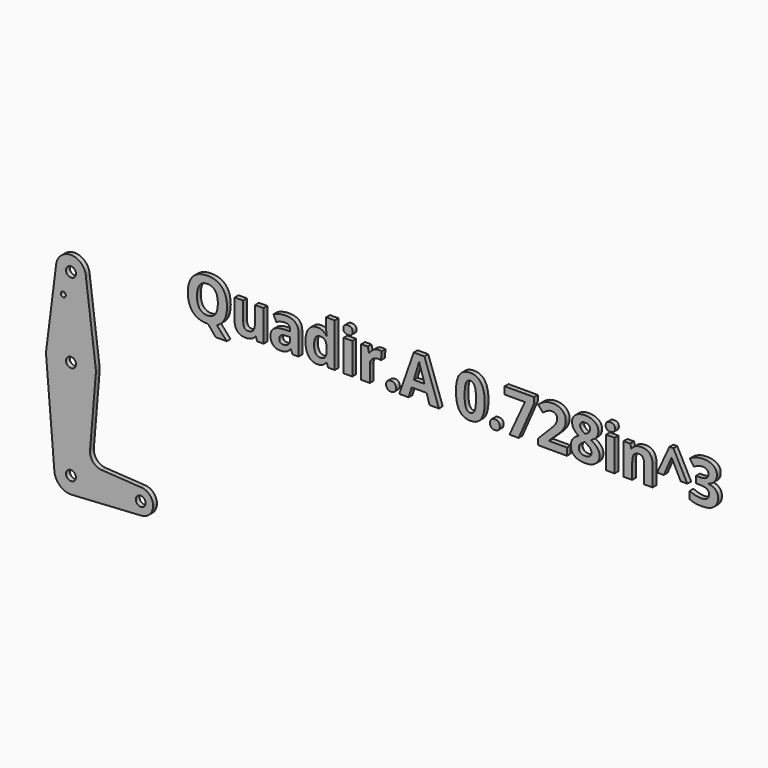
from build123d import *

# Parameters (mm, degrees)
F0_R         = 3.175
F0_R_2       = 1.5875
F0_R_3       = 3.1332260433
F0_R_4       = 3.1320796643
F0_TEXT_SIZE = 36.6663353311
F1_DEPTH     = 3.048


# Not quite as in the source:
# - Text() gives the source's letters only with a copy of the font that has no kerning and outlines rounded to 1/6400 em; it was checked with that copy


with BuildPart() as f1:
    # F0 (on Front) → F1 (new body)
    with BuildSketch(Plane.XZ):
        with BuildLine():
            ThreePointArc((-39.3125587135, 78.4643656567), (-30.4570816653, 67.7700037653), (-20.3369320583, 77.2763922459))
            ThreePointArc((-20.3369320583, 77.2763922459), (-20.3403427357, 77.5312682375), (-20.3505723252, 77.7859616989))
            ThreePointArc((-20.3505723252, 77.7859616989), (-29.521373533, 86.7953021042), (-39.3125587135, 78.4643656567))
        make_face()
        with Locations((-29.8619320583, 77.2763922459)):
            Circle(F0_R, mode=Mode.SUBTRACT)
        with BuildLine():
            ThreePointArc((-20.3505723252, 77.7859616989), (-20.3403427357, 77.5312682375), (-20.3369320583, 77.2763922459))
            ThreePointArc((-20.3369320583, 77.2763922459), (-30.4570816653, 67.7700037653), (-39.3125587135, 78.4643656567))
            Line((-39.3125587135, 78.4643656567), (-45.5153906923, 29.1192804))
            ThreePointArc((-45.5153906923, 29.1192804), (-29.5330383504, 42.3479849174), (-14.1124253975, 28.468543079))
            Line((-14.1124253975, 28.468543079), (-20.3505723252, 77.7859616989))
        make_face()
        with Locations((-34.7417071462, 63.0015922459)):
            Circle(F0_R_2, mode=Mode.SUBTRACT)
        with BuildLine():
            Line((-14.1124253975, 24.4842414128), (-14.1124253975, 28.468543079))
            ThreePointArc((-14.1124253975, 28.468543079), (-29.5330383504, 42.3479849174), (-45.5153906923, 29.1192804))
            Line((-45.5153906923, 29.1192804), (-45.6824995011, 27.7898878824))
            ThreePointArc((-45.6824995011, 27.7898878824), (-45.7369320583, 26.4763922459), (-45.6824995011, 25.1628966095))
            ThreePointArc((-45.6824995011, 25.1628966095), (-30.2031147479, 10.6050589884), (-14.1124253975, 24.4842414128))
        make_face()
        with Locations((-29.8619320583, 26.4763922459)):
            Circle(F0_R, mode=Mode.SUBTRACT)
        with BuildLine():
            ThreePointArc((-13.9869320583, 26.4763922459), (-14.0183364557, 27.4744420342), (-14.1124253975, 28.468543079))
            Line((-14.1124253975, 28.468543079), (-14.1124253975, 24.4842414128))
            ThreePointArc((-14.1124253975, 24.4842414128), (-14.0183364557, 25.4783424576), (-13.9869320583, 26.4763922459))
        make_face()
        with BuildLine():
            Line((-45.6824995011, 27.7898878824), (-45.5153906923, 29.1192804))
            ThreePointArc((-45.5153906923, 29.1192804), (-45.6129764836, 28.4563479305), (-45.6824995011, 27.7898878824))
        make_face()
        with BuildLine():
            Line((-17.6998397607, -18.9681708504), (-14.1124253975, 24.4842414128))
            ThreePointArc((-14.1124253975, 24.4842414128), (-30.2031147479, 10.6050589884), (-45.6824995011, 25.1628966095))
            Line((-45.6824995011, 25.1628966095), (-40.53226543, -36.8697612897))
            ThreePointArc((-40.53226543, -36.8697612897), (-29.7850068275, -26.3524426112), (-19.1904896536, -37.0236077541))
            ThreePointArc((-19.1904896536, -37.0236077541), (-21.9201856875, -44.1516051993), (-28.7127914479, -47.6329978805))
            Line((-28.7127914479, -47.6329978805), (15.0742024143, -44.946207045))
            ThreePointArc((15.0742024143, -44.946207045), (6.6542939935, -37.2667891455), (14.5880679417, -29.0861077541))
            Line((14.5880679417, -29.0861077541), (-10.264659502, -27.5575155059))
            ThreePointArc((-10.264659502, -27.5575155059), (-15.7875639167, -24.8255744077), (-17.6998397607, -18.9681708504))
        make_face()
        with BuildLine():
            ThreePointArc((-19.1904896536, -37.0236077541), (-29.7850068275, -26.3524426112), (-40.53226543, -36.8697612897))
            ThreePointArc((-40.53226543, -36.8697612897), (-37.4068108686, -44.5704273978), (-29.7053411314, -47.6939012027))
            Line((-29.7053411314, -47.6939012027), (-28.7127914479, -47.6329978805))
            ThreePointArc((-28.7127914479, -47.6329978805), (-21.9201856875, -44.1516051993), (-19.1904896536, -37.0236077541))
        make_face()
        with Locations((-29.8619320583, -37.0236077541)):
            Circle(F0_R_3, mode=Mode.SUBTRACT)
        with BuildLine():
            Line((-28.7127914479, -47.6329978805), (-29.7053411314, -47.6939012027))
            ThreePointArc((-29.7053411314, -47.6939012027), (-29.208356496, -47.6750171436), (-28.7127914479, -47.6329978805))
        make_face()
        with BuildLine():
            ThreePointArc((22.5255679417, -37.0236077541), (20.2007280174, -31.4109476784), (14.5880679417, -29.0861077541))
            ThreePointArc((14.5880679417, -29.0861077541), (6.6542939935, -37.2667891455), (15.0742024143, -44.946207045))
            ThreePointArc((15.0742024143, -44.946207045), (20.3700485118, -42.4616779023), (22.5255679417, -37.0236077541))
        make_face()
        with Locations((14.5880679417, -37.0236077541)):
            Circle(F0_R_4, mode=Mode.SUBTRACT)
        with Locations((42.5469912589, 76.8721103668)):
            Text('Quadir.A 0.728in^3', F0_TEXT_SIZE, font='Open Sans', font_style=FontStyle.BOLD, text_align=(TextAlign.LEFT, TextAlign.BOTTOM))
    extrude(amount=F1_DEPTH)


solid = f1.part
